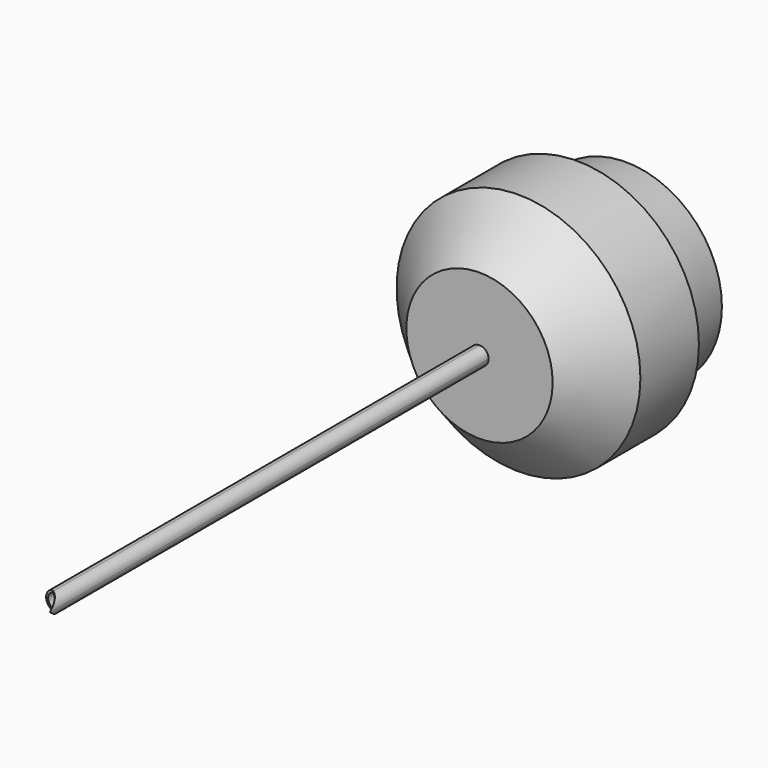
from build123d import *

# Parameters (mm, degrees)
F0_R      = 21.59
F1_DEPTH  = 12.7
F2_R      = 25.4
F3_DEPTH  = 25.4
F4_SIZE   = 10.16
F5_W      = 3.81
F5_H      = 3.81
F6_DEPTH  = 114.3
F8_D      = 7.62
F9_R      = 1.9049
F11_D     = 38.1
F11_DEPTH = 25.4
F11_TIP   = 11.4463947925
F13_D     = 2.921
F13_DEPTH = 254
F13_START = 35.9688379
F13_TIP   = 0.8775569341
F14_SIZE2 = 1.559354
F14_SIZE  = 12.69999


# Not quite as in the source:
# - a fillet or chamfer is up to 0.001 mm smaller than in the source, because OpenCascade refuses the exact size


with BuildPart() as f1:
    # F0 (on Front) → F1 (new body)
    with BuildSketch(Plane.XZ):
        Circle(F0_R)
    extrude(amount=F1_DEPTH)

    # F2 (on face) → F3 (join)
    with BuildSketch(Plane.XZ.offset(12.7)):
        Circle(F2_R)
    extrude(amount=F3_DEPTH)

    # F4
    f4_edges = [f1.edges().sort_by_distance(p)[0] for p in [
        (-25.4, -38.1, 0),
    ]]
    chamfer(f4_edges, length=F4_SIZE)

    # F5 (on face) → F6 (join)
    with BuildSketch(Plane.XZ.offset(38.1)):
        Rectangle(F5_W, F5_H)
    extrude(amount=F6_DEPTH)

    # F8 (through all)
    with Locations(Plane.XY.offset(1.905)):
        with Locations((-1.905, -152.4)):
            Hole(F8_D / 2)

    # F9 (radius 1.905 in the source; OpenCascade refuses exactly that, so slightly less here)
    f9_edges = [f1.edges().sort_by_distance(p)[0] for p in [
        (1.905, -95.25, -1.905),
        (1.905, -95.25, 1.905),
        (-1.905, -93.345, 1.905),
        (-1.905, -93.345, -1.905),
    ]]
    fillet(f9_edges, radius=F9_R)

    # F11
    with Locations(Plane(origin=(0, 0, 0), x_dir=(-1, 0, 0), z_dir=(0, 1, 0))):
        with Locations((0, 0)):
            Hole(F11_D / 2, depth=F11_DEPTH)
            with Locations((0, 0, -(F11_DEPTH + F11_TIP / 2))):  # 118° drill point
                Cone(0, F11_D / 2, F11_TIP, mode=Mode.SUBTRACT)

    # F13
    # its depths count from where the whole tool has entered the part; down to there all is cleared
    with Locations(Plane(origin=(0, 0, 0), x_dir=(1, 0, 0), z_dir=(0, 1, 0)).offset(-F13_START)):
        with Locations((0, 0)):
            Hole(F13_D / 2, depth=F13_DEPTH)
            with Locations((0, 0, -(F13_DEPTH + F13_TIP / 2))):  # 118° drill point
                Cone(0, F13_D / 2, F13_TIP, mode=Mode.SUBTRACT)

    # F14 (size 12.7 and 1.5593639235 in the source; OpenCascade refuses exactly that, so slightly less here)
    f14_edges = [f1.edges().sort_by_distance(p)[0] for p in [
        (-21.59, 0, 0),
    ]]
    f14_side = f1.faces().sort_by_distance((-21.59, -6.35, 0))[0]
    chamfer(f14_edges, length=F14_SIZE, length2=F14_SIZE2, reference=f14_side)


solid = f1.part
